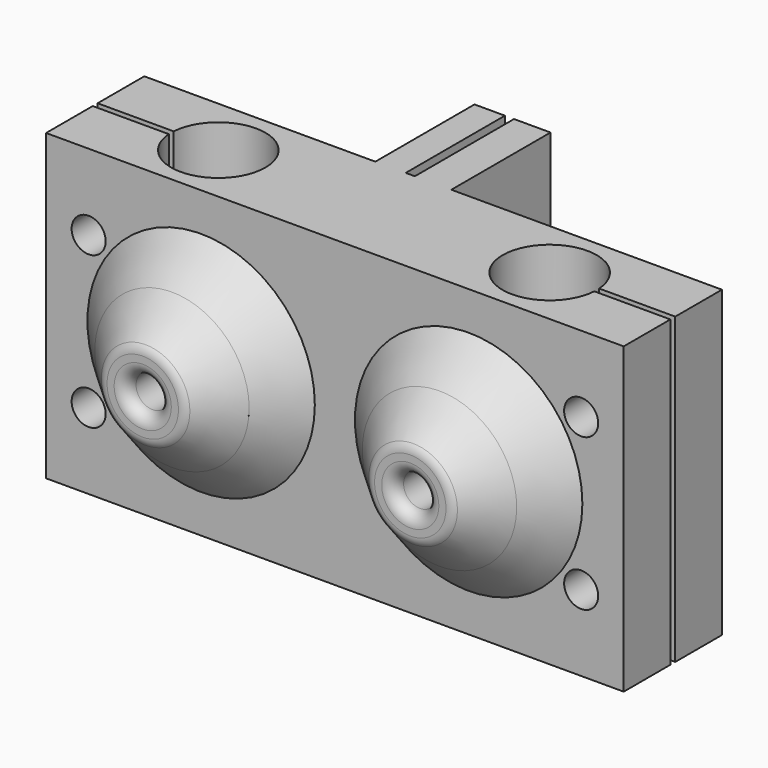
from build123d import *

# Parameters (mm, degrees)
F0_W     = 5
F0_H     = 20.3830654012
F0_W_2   = 3
F1_DEPTH = 50
F2_R     = 2.7
F3_DEPTH = 25
F4_R     = 12.7
F4_R_2   = 2.7
F5_DEPTH = 12
F6_SIZE  = 5.99999
F4_R_3   = 2.8
F7_DEPTH = 25
F8_R     = 2


# Not quite as in the source:
# - a fillet or chamfer is up to 0.001 mm smaller than in the source, because OpenCascade refuses the exact size


with BuildPart() as f1:
    # F0 (on Top) → F1 (new body)
    with BuildSketch(Plane.XY):
        with BuildLine():
            ThreePointArc((-34.9838541491, 0.5), (-26.9998696897, 7.7459624856), (-19.5, 0))
            ThreePointArc((-19.5, 0), (-26.9998696897, -7.7459624856), (-34.9838541491, -0.5))
            Line((-34.9838541491, -0.5), (-47.5, -0.5))
            Line((-47.5, -0.5), (-47.5, -10.0949762179))
            Line((-47.5, -10.0949762179), (47.5, -10.0949762179))
            Line((47.5, -10.0949762179), (47.5, -0.5))
            Line((47.5, -0.5), (34.9838541491, -0.5))
            ThreePointArc((34.9838541491, -0.5), (19.5, 0), (34.9838541491, 0.5))
            Line((34.9838541491, 0.5), (47.5, 0.5))
            Line((47.5, 0.5), (47.5, 10.0949762179))
            Line((47.5, 10.0949762179), (9.5, 10.0949762179))
            Line((9.5, 10.0949762179), (4.5, 10.0949762179))
            Line((4.5, 10.0949762179), (3, 10.0949762179))
            Line((3, 10.0949762179), (0, 10.0949762179))
            Line((0, 10.0949762179), (-3, 10.0949762179))
            Line((-3, 10.0949762179), (-4.5, 10.0949762179))
            Line((-4.5, 10.0949762179), (-9.5, 10.0949762179))
            Line((-9.5, 10.0949762179), (-47.5, 10.0949762179))
            Line((-47.5, 10.0949762179), (-47.5, 0.5))
            Line((-47.5, 0.5), (-34.9838541491, 0.5))
        make_face()
        with Locations((-7, 20.2865089185)):
            Rectangle(F0_W, F0_H)
        with Locations((-1.5, 20.2865089185)):
            Rectangle(F0_W_2, F0_H)
        with Locations((1.5, 20.2865089185)):
            Rectangle(F0_W_2, F0_H)
    extrude(amount=F1_DEPTH)

    # F2 (on face) → F3 (cut)
    with BuildSketch(Plane.YZ.offset(3)):
        with Locations((20.2865089185, 37.5)):
            Circle(F2_R)
        with Locations((20.2865089185, 12.5)):
            Circle(F2_R)
    extrude(amount=-F3_DEPTH, mode=Mode.SUBTRACT)

    # F4 (on face) → F5 (join)
    with BuildSketch(Plane.XZ.offset(10.0949762179)):
        with Locations((-22, 25)):
            Circle(F4_R)
        with Locations((-22, 25)):
            Circle(F4_R_2, mode=Mode.SUBTRACT)
        with Locations((22, 25)):
            Circle(F4_R)
        with Locations((22, 25)):
            Circle(F4_R_2, mode=Mode.SUBTRACT)
    extrude(amount=F5_DEPTH)

    # F6 (size 6 in the source; OpenCascade refuses exactly that, so slightly less here)
    f6_edges = [f1.edges().sort_by_distance(p)[0] for p in [
        (-34.7, -10.094976, 25),
        (-34.7, -22.094976, 25),
        (9.3, -22.094976, 25),
        (9.3, -10.094976, 25),
    ]]
    chamfer(f6_edges, length=F6_SIZE)

    # F4 (on face) → F7 (cut)
    with BuildSketch(Plane.XZ.offset(10.0949762179)):
        with Locations((-40.5, 37.5)):
            Circle(F4_R_3)
        with Locations((-40.5, 12.5)):
            Circle(F4_R_3)
        with Locations((40.5, 37.5)):
            Circle(F4_R_3)
        with Locations((40.5, 12.5)):
            Circle(F4_R_3)
    extrude(amount=-F7_DEPTH, mode=Mode.SUBTRACT)

    # F8
    f8_edges = [f1.edges().sort_by_distance(p)[0] for p in [
        (-28.70001, -22.094976, 25),
        (-24.7, -22.094976, 25),
        (15.29999, -22.094976, 25),
        (19.3, -22.094976, 25),
    ]]
    fillet(f8_edges, radius=F8_R)


solid = f1.part
